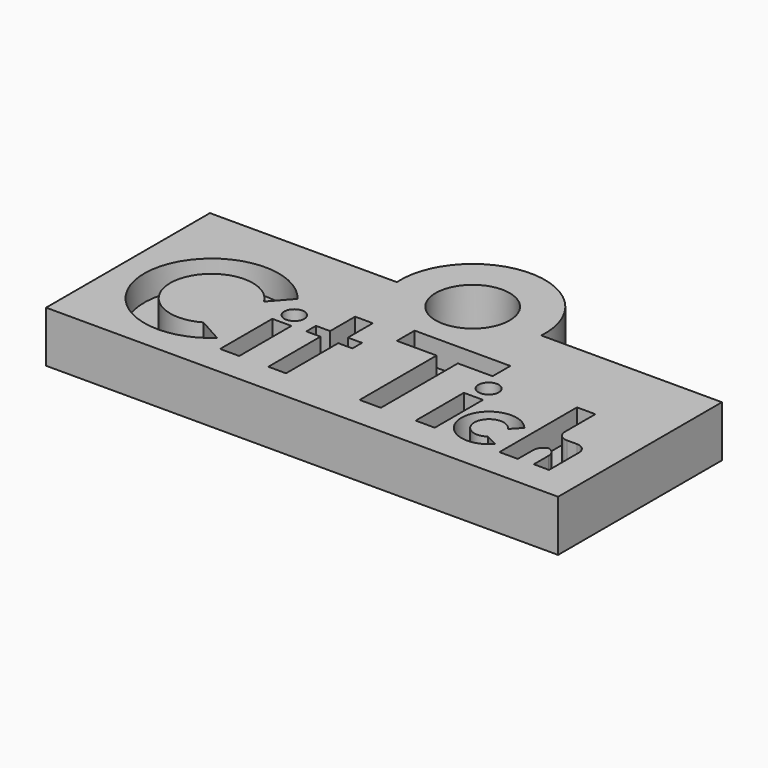
from build123d import *

# Parameters (mm, degrees)
F0_R     = 4.5926712991
F1_DEPTH = 6.35
F2_W     = 2.3739238567
F2_H     = 8.0889270103
F2_W_2   = 2.3739274609
F2_H_2   = 7.4734649694
F2_R     = 1.2680453983
F2_R_2   = 1.2379691671
F3_DEPTH = 3.175


# Not quite as in the source:
# - a length typed as a fraction of an inch, garbled in the dataset ("3 / 203.2 mm" for 3/8 in), is restored


with BuildPart() as f1:
    # F0 (on Top) → F1 (new body)
    with BuildSketch(Plane.XY):
        with BuildLine():
            Line((-63.5, 0), (0, 0))
            Line((0, 0), (0, 25.4))
            Line((0, 25.4), (-22.4021356553, 25.4))
            ThreePointArc((-22.4021356553, 25.4), (-31.3605917618, 34.9369900473), (-40.3190478683, 25.4))
            Line((-40.3190478683, 25.4), (-63.5, 25.4))
            Line((-63.5, 25.4), (-63.5, 0))
        make_face()
        with Locations((-31.3605917618, 25.960986396)):
            Circle(F0_R, mode=Mode.SUBTRACT)
    extrude(amount=F1_DEPTH)

    # F2 (on face) → F3 (cut)
    with BuildSketch(Plane.XY.offset(6.35)):
        with BuildLine():
            Line((-47.8143577063, 14.1739739048), (-45.6251816468, 16.6567004661))
            ThreePointArc((-45.6251816468, 16.6567004661), (-60.5221954701, 12.262678636), (-46.5953443626, 5.3872683266))
            Line((-46.5953443626, 5.3872683266), (-49.6666999843, 7.1012593313))
            ThreePointArc((-49.6666999843, 7.1012593313), (-57.1721052058, 12.8458444774), (-47.8143577063, 14.1739739048))
        make_face()
        Polygon((-20.7504647221, 18.5370575163), (-32.6200858075, 18.5370575163), (-32.6200858075, 15.7841322933), (-27.6963894798, 15.7841322933), (-27.6963894798, 3.8538966697), (-25.0586963057, 3.8538966697), (-25.0586963057, 15.7841322933), (-20.7504647221, 15.7841322933), align=None)
        with BuildLine():
            Line((-8.0016118277, 15.7841322933), (-10.2876118277, 15.7841322933))
            Line((-10.2876118277, 15.7841322933), (-10.2876118277, 3.7659732636))
            Line((-10.2876118277, 3.7659732636), (-8.0016118277, 3.7659732636))
            Line((-8.0016118277, 3.7659732636), (-8.0016118277, 6.1422445658))
            ThreePointArc((-8.0016118277, 6.1422445658), (-7.7348762924, 6.9209360412), (-7.0467135382, 7.3725335205))
            ThreePointArc((-7.0467135382, 7.3725335205), (-6.358550784, 6.9209360412), (-6.0918152487, 6.1422445658))
            Line((-6.0918152487, 6.1422445658), (-6.0918152487, 3.8510074993))
            Line((-6.0918152487, 3.8510074993), (-4.2027005772, 3.8510074993))
            Line((-4.2027005772, 3.8510074993), (-4.2027005772, 8.5050527784))
            ThreePointArc((-4.2027005772, 8.5050527784), (-4.5746749651, 9.4030783905), (-5.4727005772, 9.7750527784))
            Line((-5.4727005772, 9.7750527784), (-6.7316118277, 9.7750527784))
            ThreePointArc((-6.7316118277, 9.7750527784), (-7.6296374398, 10.1470271663), (-8.0016118277, 11.0450527784))
            Line((-8.0016118277, 11.0450527784), (-8.0016118277, 15.7841322933))
        make_face()
        with BuildLine():
            ThreePointArc((-6.7316118277, 7.4122445658), (-6.8904089113, 7.4022776948), (-7.0467135382, 7.3725335205))
            ThreePointArc((-7.0467135382, 7.3725335205), (-7.203018165, 7.4022776948), (-7.3618152487, 7.4122445658))
            Line((-7.3618152487, 7.4122445658), (-6.7316118277, 7.4122445658))
        make_face(mode=Mode.SUBTRACT)
        Polygon((-36.7524705789, 17.2182109293), (-38.9505494254, 17.2182109293), (-38.9505494254, 13.3495927722), (-40.7090139442, 13.3495927722), (-40.7090139442, 11.8549002739), (-38.9505494254, 11.8549002739), (-38.9505494254, 3.7659732636), (-36.7524705789, 3.7659732636), (-36.7524705789, 11.8549002739), (-34.9940096642, 11.8549002739), (-34.9940096642, 13.3495927722), (-36.7524705789, 13.3495927722), align=None)
        with BuildLine():
            Line((-12.6827618144, 8.0606505512), (-11.5731045271, 9.2428652738))
            ThreePointArc((-11.5731045271, 9.2428652738), (-17.6629146287, 7.19801004), (-11.6904523614, 4.8322301544))
            Line((-11.6904523614, 4.8322301544), (-13.1890844097, 5.6123530456))
            ThreePointArc((-13.1890844097, 5.6123530456), (-16.0358025283, 7.4775754374), (-12.6827618144, 8.0606505512))
        make_face()
        with Locations((-43.7423610944, 7.8104367687)):
            Rectangle(F2_W, F2_H)
        with Locations((-19.5635009916, 7.5906291544)):
            Rectangle(F2_W_2, F2_H_2)
        with Locations((-19.4316163329, 13.5254395845)):
            Circle(F2_R)
        with Locations((-43.7423610944, 13.7892089019)):
            Circle(F2_R_2)
        with BuildLine():
            ThreePointArc((-7.3618152487, 7.4122445658), (-7.203018165, 7.4022776948), (-7.0467135382, 7.3725335205))
            ThreePointArc((-7.0467135382, 7.3725335205), (-6.8904089113, 7.4022776948), (-6.7316118277, 7.4122445658))
            Line((-6.7316118277, 7.4122445658), (-7.3618152487, 7.4122445658))
        make_face()
    extrude(amount=-F3_DEPTH, mode=Mode.SUBTRACT)


solid = f1.part
